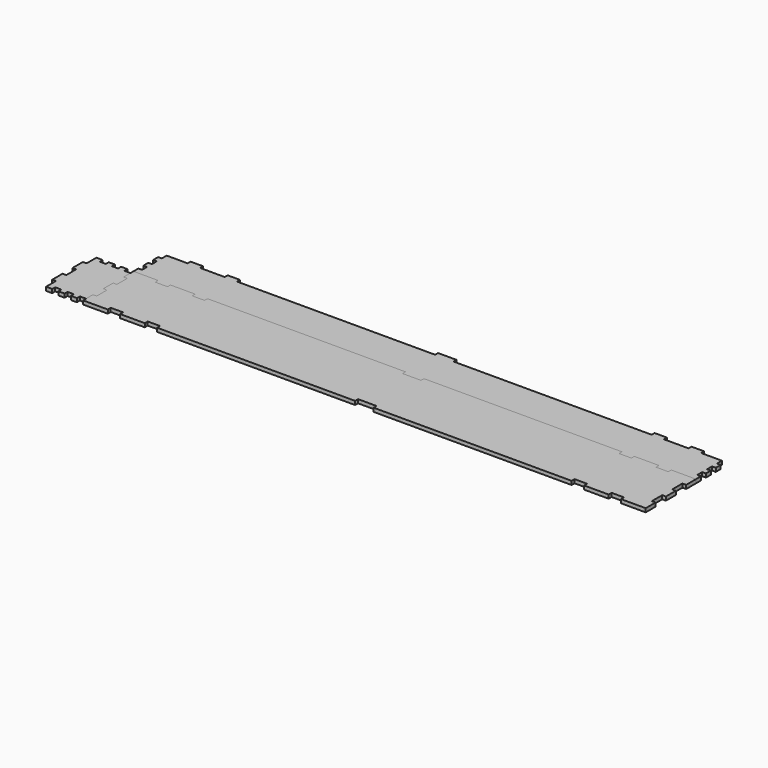
from build123d import *

# Parameters (mm, degrees)
F2_DEPTH = 3
F1_R     = 2.5
F1_R_2   = 3.5
F3_DEPTH = 3
F4_DEPTH = 3
F5_DEPTH = 3
F6_DEPTH = 3
F9_DEPTH = 3


# Not quite as in the source:
# - a feature names something its author has since deleted; it is built from what else it names


with BuildPart() as f2:
    # F1 (on Top) → F2 (new body)
    with BuildSketch(Plane.XY):
        Polygon((-228, 15.5), (-228, 22.5), (-233, 22.5), (-233, 25.5), (-238, 25.5), (-238, 22.5), (-243, 22.5), (-243, 25.5), (-248, 25.5), (-248, 22.5), (-253, 22.5), (-253, 25.5), (-258, 25.5), (-258, 15.5), (-261, 15.5), (-261, 5), (-258, 5), (-258, 0), (-258, -5), (-261, -5), (-261, -15.5), (-258, -15.5), (-258, -25.5), (-253, -25.5), (-253, -22.5), (-248, -22.5), (-248, -25.5), (-243, -25.5), (-243, -22.5), (-238, -22.5), (-238, -25.5), (-233, -25.5), (-233, -22.5), (-228, -22.5), (-228, -15.5), (-225, -15.5), (-225, -5), (-228, -5), (-228, 5), (-225, 5), (-225, 15.5), align=None)
    extrude(amount=F2_DEPTH)


with BuildPart() as f3:
    # F1 (on Top) → F3 (new body)
    with BuildSketch(Plane.XY):
        Polygon((-208, 25.5), (-228, 25.5), (-228, 22.5), (-228, 15.5), (-225, 15.5), (-225, 5), (-228, 5), (-228, -5), (-225, -5), (-225, -15.5), (-228, -15.5), (-228, -22.5), (-228, -25.5), (-208, -25.5), (-208, -22.5), (-198, -22.5), (-198, -25.5), (-178, -25.5), (-178, -22.5), (-168, -22.5), (-168, -25.5), (-7.5, -25.5), (-7.5, -22.5), (7.5, -22.5), (7.5, -25.5), (168, -25.5), (168, -22.5), (178, -22.5), (178, -25.5), (198, -25.5), (198, -22.5), (208, -22.5), (208, -25.5), (228, -25.5), (228, -15.5), (225, -15.5), (225, -5), (228, -5), (228, 5), (225, 5), (225, 15.5), (228, 15.5), (228, 25.5), (208, 25.5), (208, 22.5), (198, 22.5), (198, 25.5), (178, 25.5), (178, 22.5), (168, 22.5), (168, 25.5), (7.5, 25.5), (7.5, 22.5), (-7.5, 22.5), (-7.5, 25.5), (-168, 25.5), (-168, 22.5), (-178, 22.5), (-178, 25.5), (-198, 25.5), (-198, 22.5), (-208, 22.5), align=None)
        with Locations((-189.0112310648, -13.972199522)):
            Circle(F1_R, mode=Mode.SUBTRACT)
        with Locations((-198.1403976679, -9.9060386419)):
            Circle(F1_R, mode=Mode.SUBTRACT)
        with Locations((-179.8765510321, -9.9060386419)):
            Circle(F1_R, mode=Mode.SUBTRACT)
        with Locations((-189.0112310648, -5.7085431231)):
            Circle(F1_R, mode=Mode.SUBTRACT)
        with Locations((-198.1403976679, 0)):
            Circle(F1_R_2, mode=Mode.SUBTRACT)
        with Locations((-179.8765510321, 0)):
            Circle(F1_R_2, mode=Mode.SUBTRACT)
        with Locations((-189.0112310648, 5.7085431231)):
            Circle(F1_R, mode=Mode.SUBTRACT)
        with Locations((-198.1403976679, 9.9060386419)):
            Circle(F1_R, mode=Mode.SUBTRACT)
        with Locations((-179.8765510321, 9.9060386419)):
            Circle(F1_R, mode=Mode.SUBTRACT)
        with Locations((-189.0112310648, 13.972199522)):
            Circle(F1_R, mode=Mode.SUBTRACT)
        Polygon((-228, 15.5), (-228, 22.5), (-233, 22.5), (-233, 25.5), (-238, 25.5), (-238, 22.5), (-243, 22.5), (-243, 25.5), (-248, 25.5), (-248, 22.5), (-253, 22.5), (-253, 25.5), (-258, 25.5), (-258, 15.5), (-261, 15.5), (-261, 5), (-258, 5), (-258, 0), (-258, -5), (-261, -5), (-261, -15.5), (-258, -15.5), (-258, -25.5), (-253, -25.5), (-253, -22.5), (-248, -22.5), (-248, -25.5), (-243, -25.5), (-243, -22.5), (-238, -22.5), (-238, -25.5), (-233, -25.5), (-233, -22.5), (-228, -22.5), (-228, -15.5), (-225, -15.5), (-225, -5), (-228, -5), (-228, 5), (-225, 5), (-225, 15.5), align=None)
    extrude(amount=F3_DEPTH)


with BuildPart() as f4:
    # F1 (on Top) → F4 (new body)
    with BuildSketch(Plane.XY):
        Polygon((-208, 25.5), (-228, 25.5), (-228, 22.5), (-228, 15.5), (-225, 15.5), (-225, 5), (-228, 5), (-228, -5), (-225, -5), (-225, -15.5), (-228, -15.5), (-228, -22.5), (-228, -25.5), (-208, -25.5), (-208, -22.5), (-198, -22.5), (-198, -25.5), (-178, -25.5), (-178, -22.5), (-168, -22.5), (-168, -25.5), (-7.5, -25.5), (-7.5, -22.5), (7.5, -22.5), (7.5, -25.5), (168, -25.5), (168, -22.5), (178, -22.5), (178, -25.5), (198, -25.5), (198, -22.5), (208, -22.5), (208, -25.5), (228, -25.5), (228, -15.5), (225, -15.5), (225, -5), (228, -5), (228, 5), (225, 5), (225, 15.5), (228, 15.5), (228, 25.5), (208, 25.5), (208, 22.5), (198, 22.5), (198, 25.5), (178, 25.5), (178, 22.5), (168, 22.5), (168, 25.5), (7.5, 25.5), (7.5, 22.5), (-7.5, 22.5), (-7.5, 25.5), (-168, 25.5), (-168, 22.5), (-178, 22.5), (-178, 25.5), (-198, 25.5), (-198, 22.5), (-208, 22.5), align=None)
        with Locations((-189.0112310648, -13.972199522)):
            Circle(F1_R, mode=Mode.SUBTRACT)
        with Locations((-198.1403976679, -9.9060386419)):
            Circle(F1_R, mode=Mode.SUBTRACT)
        with Locations((-179.8765510321, -9.9060386419)):
            Circle(F1_R, mode=Mode.SUBTRACT)
        with Locations((-189.0112310648, -5.7085431231)):
            Circle(F1_R, mode=Mode.SUBTRACT)
        with Locations((-198.1403976679, 0)):
            Circle(F1_R_2, mode=Mode.SUBTRACT)
        with Locations((-179.8765510321, 0)):
            Circle(F1_R_2, mode=Mode.SUBTRACT)
        with Locations((-189.0112310648, 5.7085431231)):
            Circle(F1_R, mode=Mode.SUBTRACT)
        with Locations((-198.1403976679, 9.9060386419)):
            Circle(F1_R, mode=Mode.SUBTRACT)
        with Locations((-179.8765510321, 9.9060386419)):
            Circle(F1_R, mode=Mode.SUBTRACT)
        with Locations((-189.0112310648, 13.972199522)):
            Circle(F1_R, mode=Mode.SUBTRACT)
    extrude(amount=F4_DEPTH)


with BuildPart() as f5:
    # F1 (on Top) → F5 (new body)
    with BuildSketch(Plane.XY):
        Polygon((-228, 30.5), (-228, 25.5), (-208, 25.5), (-208, 22.5), (-198, 22.5), (-198, 25.5), (-178, 25.5), (-178, 22.5), (-168, 22.5), (-168, 25.5), (-7.5, 25.5), (-7.5, 22.5), (7.5, 22.5), (7.5, 25.5), (168, 25.5), (168, 22.5), (178, 22.5), (178, 25.5), (198, 25.5), (198, 22.5), (208, 22.5), (208, 25.5), (228, 25.5), (228, 30.5), (225, 30.5), (225, 35.5), (228, 35.5), (228, 40.5), (225, 40.5), (225, 45.5), (228, 45.5), (228, 50.5), (225, 50.5), (225, 55.5), (208, 55.5), (208, 58.5), (198, 58.5), (198, 55.5), (178, 55.5), (178, 58.5), (168, 58.5), (168, 55.5), (7.5, 55.5), (7.5, 58.5), (-7.5, 58.5), (-7.5, 55.5), (-168, 55.5), (-168, 58.5), (-178, 58.5), (-178, 55.5), (-198, 55.5), (-198, 58.5), (-208, 58.5), (-208, 55.5), (-225, 55.5), (-225, 50.5), (-228, 50.5), (-228, 45.5), (-225, 45.5), (-225, 40.5), (-228, 40.5), (-228, 35.5), (-225, 35.5), (-225, 30.5), align=None)
    extrude(amount=F5_DEPTH)


with BuildPart() as f6:
    # F1 (on Top) → F6 (new body)
    with BuildSketch(Plane.XY):
        Polygon((-228, 15.5), (-228, 22.5), (-233, 22.5), (-233, 25.5), (-238, 25.5), (-238, 22.5), (-243, 22.5), (-243, 25.5), (-248, 25.5), (-248, 22.5), (-253, 22.5), (-253, 25.5), (-258, 25.5), (-258, 15.5), (-261, 15.5), (-261, 5), (-258, 5), (-258, 0), (-258, -5), (-261, -5), (-261, -15.5), (-258, -15.5), (-258, -25.5), (-253, -25.5), (-253, -22.5), (-248, -22.5), (-248, -25.5), (-243, -25.5), (-243, -22.5), (-238, -22.5), (-238, -25.5), (-233, -25.5), (-233, -22.5), (-228, -22.5), (-228, -15.5), (-225, -15.5), (-225, -5), (-228, -5), (-228, 5), (-225, 5), (-225, 15.5), align=None)
    extrude(amount=F6_DEPTH)


with BuildPart() as f9:
    # F1 (on Top) → F9 (new body)
    with BuildSketch(Plane.XY):
        Polygon((-208, 25.5), (-228, 25.5), (-228, 22.5), (-228, 15.5), (-225, 15.5), (-225, 5), (-228, 5), (-228, -5), (-225, -5), (-225, -15.5), (-228, -15.5), (-228, -22.5), (-228, -25.5), (-208, -25.5), (-208, -22.5), (-198, -22.5), (-198, -25.5), (-178, -25.5), (-178, -22.5), (-168, -22.5), (-168, -25.5), (-7.5, -25.5), (-7.5, -22.5), (7.5, -22.5), (7.5, -25.5), (168, -25.5), (168, -22.5), (178, -22.5), (178, -25.5), (198, -25.5), (198, -22.5), (208, -22.5), (208, -25.5), (228, -25.5), (228, -15.5), (225, -15.5), (225, -5), (228, -5), (228, 5), (225, 5), (225, 15.5), (228, 15.5), (228, 25.5), (208, 25.5), (208, 22.5), (198, 22.5), (198, 25.5), (178, 25.5), (178, 22.5), (168, 22.5), (168, 25.5), (7.5, 25.5), (7.5, 22.5), (-7.5, 22.5), (-7.5, 25.5), (-168, 25.5), (-168, 22.5), (-178, 22.5), (-178, 25.5), (-198, 25.5), (-198, 22.5), (-208, 22.5), align=None)
        with Locations((-189.0112310648, -13.972199522)):
            Circle(F1_R, mode=Mode.SUBTRACT)
        with Locations((-198.1403976679, -9.9060386419)):
            Circle(F1_R, mode=Mode.SUBTRACT)
        with Locations((-179.8765510321, -9.9060386419)):
            Circle(F1_R, mode=Mode.SUBTRACT)
        with Locations((-189.0112310648, -5.7085431231)):
            Circle(F1_R, mode=Mode.SUBTRACT)
        with Locations((-198.1403976679, 0)):
            Circle(F1_R_2, mode=Mode.SUBTRACT)
        with Locations((-179.8765510321, 0)):
            Circle(F1_R_2, mode=Mode.SUBTRACT)
        with Locations((-189.0112310648, 5.7085431231)):
            Circle(F1_R, mode=Mode.SUBTRACT)
        with Locations((-198.1403976679, 9.9060386419)):
            Circle(F1_R, mode=Mode.SUBTRACT)
        with Locations((-179.8765510321, 9.9060386419)):
            Circle(F1_R, mode=Mode.SUBTRACT)
        with Locations((-189.0112310648, 13.972199522)):
            Circle(F1_R, mode=Mode.SUBTRACT)
        with Locations((-179.8765510321, -9.9060386419)):
            Circle(F1_R)
        with Locations((-179.8765510321, 0)):
            Circle(F1_R_2)
        with Locations((-179.8765510321, 9.9060386419)):
            Circle(F1_R)
        with Locations((-189.0112310648, 5.7085431231)):
            Circle(F1_R)
        with Locations((-189.0112310648, -5.7085431231)):
            Circle(F1_R)
        with Locations((-189.0112310648, -13.972199522)):
            Circle(F1_R)
        with Locations((-198.1403976679, -9.9060386419)):
            Circle(F1_R)
        with Locations((-198.1403976679, 0)):
            Circle(F1_R_2)
        with Locations((-198.1403976679, 9.9060386419)):
            Circle(F1_R)
        with Locations((-189.0112310648, 13.972199522)):
            Circle(F1_R)
    extrude(amount=F9_DEPTH)


solid = Compound([f4.part, f5.part, f6.part, f9.part])
